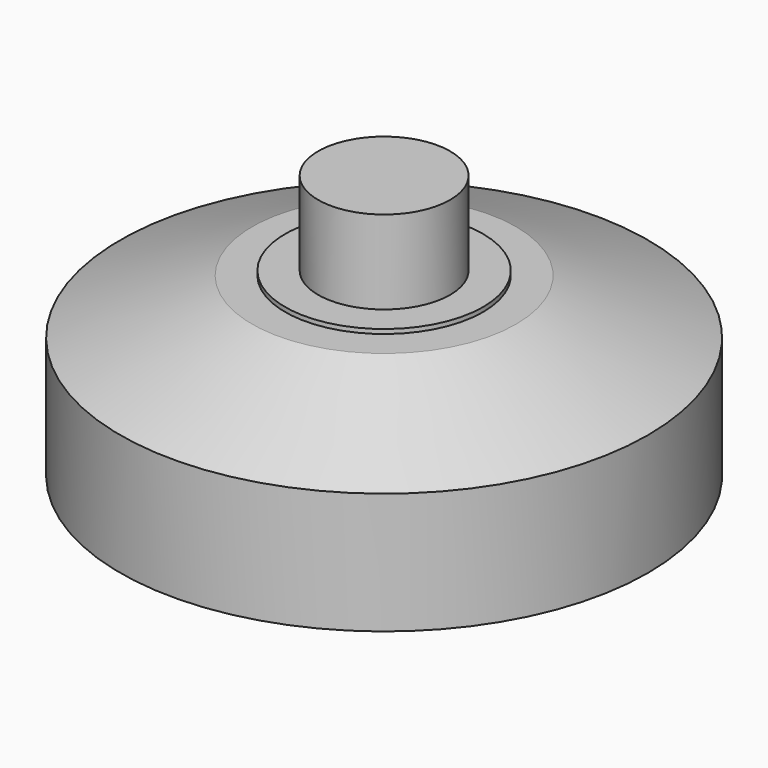
from build123d import *

# Parameters (mm, degrees)
F0_R     = 1.5
F1_DEPTH = 6
F0_R_2   = 2.25
F2_DEPTH = 4.1
F0_R_3   = 6
F3_DEPTH = 4
F4_SIZE  = 1


# Not quite as in the source:
# - a fillet or chamfer that OpenCascade refuses, or shapes differently, is made with other operations: its cross-section is extruded or revolved along the edge and cut away or added


with BuildPart() as f1:
    # F0 (on Top) → F1 (new body)
    with BuildSketch(Plane.XY):
        Circle(F0_R)
    extrude(amount=F1_DEPTH)

    # F0 (on Top) → F2 (join)
    with BuildSketch(Plane.XY):
        Circle(F0_R_2)
        Circle(F0_R, mode=Mode.SUBTRACT)
    extrude(amount=F2_DEPTH)

    # F0 (on Top) → F3 (join)
    with BuildSketch(Plane.XY):
        Circle(F0_R_3)
        Circle(F0_R_2, mode=Mode.SUBTRACT)
    extrude(amount=F3_DEPTH)

    # F4
    f4_edges = [f1.edges().sort_by_distance(p)[0] for p in [
        (-6, 0, 4),
    ]]
    chamfer(f4_edges, length=F4_SIZE)

    # F5: chamfer of 2 on 1 edges, made by hand

    # F5_s1 → F5_t2 (revolve, cut)
    with BuildSketch(Plane.XZ):
        Polygon((3, 4), (6.4142135624, 2.5857864376), (5, 4), align=None)
    revolve(axis=Axis((0, 0, 4), (0, 0, 1)), mode=Mode.SUBTRACT)


solid = f1.part
